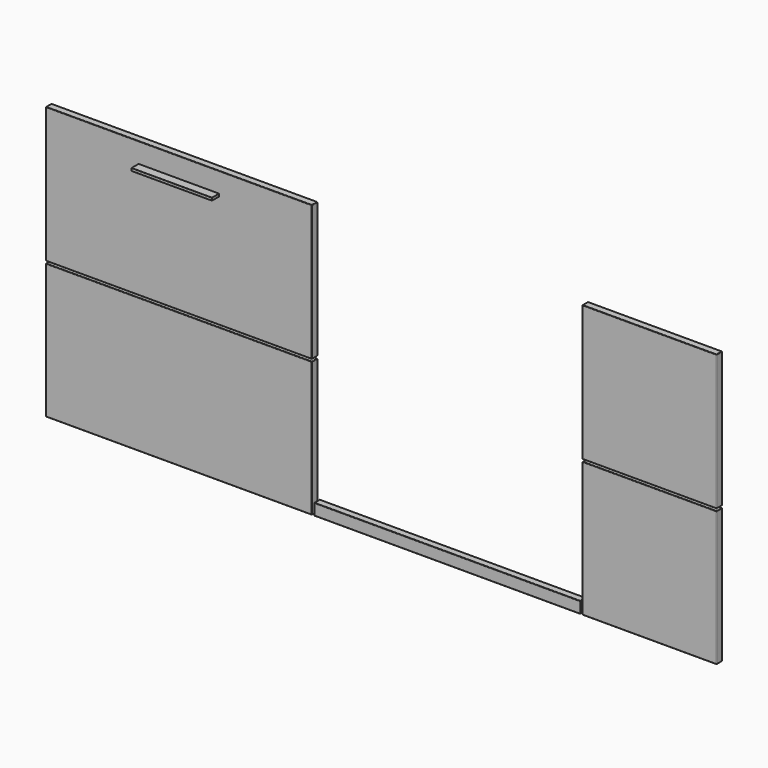
from build123d import *

# Parameters (mm, degrees)
F0_W     = 381
F0_H     = 774.7
F1_DEPTH = 19.05
F0_W_2   = 755.65
F0_H_2   = 32.6746147394
F3_W     = 228.6
F3_H     = 7.62
F4_DEPTH = 25.4
F5_R     = 0.3175
F6_W     = 2032
F6_H     = 6.35
F7_DEPTH = 25.4
F8_R     = 1.27
F8_2_R   = 1.27
F8_3_R   = 1.27


# Not quite as in the source:
# - a feature of the source that left no trace in its solid (it failed there, or was rolled back) is left out


with BuildPart() as f1:
    # F0 (on Front) → F1 (new body)
    with BuildSketch(Plane.XZ):
        with Locations((-190.5, 469.9)):
            Rectangle(F0_W, F0_H)
    extrude(amount=F1_DEPTH)


with BuildPart() as f1b:
    # F0 (on Front) → F1, piece 2 (new body)
    with BuildSketch(Plane.XZ):
        Polygon((-1904.895815666, 857.25), (-1904.9897383738, 82.4946576853), (-1149.3540530003, 82.4946576853), (-1149.3540530003, 82.55), (-1149.3540530003, 857.25), (-1527.1790530003, 857.25), align=None)
    extrude(amount=F1_DEPTH)


with BuildPart() as f1c:
    # F0 (on Front) → F1, piece 3 (new body)
    with BuildSketch(Plane.XZ):
        with Locations((-765.1790530003, 98.8873073697)):
            Rectangle(F0_W_2, F0_H_2)
    extrude(amount=F1_DEPTH)

    # F8#3
    f8_3_edges = [f1c.edges().sort_by_distance(p)[0] for p in [
        (-1143.004053, -9.525, 82.55),
        (-387.354053, -9.525, 82.55),
        (-765.179053, -19.05, 82.55),
        (-387.354053, -9.525, 115.224615),
        (-387.354053, -19.05, 98.887307),
        (-1143.004053, -9.525, 115.224615),
        (-765.179053, -19.05, 115.224615),
        (-1143.004053, -19.05, 98.887307),
    ]]
    fillet(f8_3_edges, radius=F8_3_R)


with BuildPart() as f4:
    # F3 (on face) → F4 (new body)
    with BuildSketch(Plane.XZ.offset(19.05)):
        with Locations((-1527.1250113088, 796.6017127037)):
            Rectangle(F3_W, F3_H)
    extrude(amount=F4_DEPTH)

    # F5
    f5_edges = [f4.edges().sort_by_distance(p)[0] for p in [
        (-1527.125011, -44.45, 792.791713),
        (-1412.825011, -44.45, 796.601713),
        (-1527.125011, -44.45, 800.411713),
        (-1641.425011, -44.45, 796.601713),
        (-1641.425011, -31.75, 800.411713),
        (-1641.425011, -31.75, 792.791713),
        (-1527.125011, -19.05, 800.411713),
        (-1641.425011, -19.05, 796.601713),
        (-1527.125011, -19.05, 792.791713),
        (-1412.825011, -31.75, 792.791713),
        (-1412.825011, -31.75, 800.411713),
        (-1412.825011, -19.05, 796.601713),
    ]]
    fillet(f5_edges, radius=F5_R)


with BuildPart() as f7_tool:
    # F6 (on face) → F7 (new body)
    with BuildSketch(Plane.XZ.offset(19.05)):
        with Locations((-895.2655443497, 468.8719840575)):
            Rectangle(F6_W, F6_H)
    extrude(amount=-F7_DEPTH)


with BuildPart() as f1_1:
    add(f1.part)

    # F7: cut by f7_tool
    add(f7_tool.part, mode=Mode.SUBTRACT)

    # F8
    f8_edges = [f1_1.edges().sort_by_distance(p)[0] for p in [
        (-381, -9.525, 472.046984),
        (-381, -9.525, 465.696984),
        (-381, -9.525, 82.55),
        (0, -9.525, 82.55),
        (-190.5, -19.05, 82.55),
        (-381, -19.05, 274.123492),
        (0, -9.525, 465.696984),
        (0, -19.05, 274.123492),
        (-190.5, -19.05, 465.696984),
        (-381, -19.05, 664.648492),
        (-381, -9.525, 857.25),
        (-190.5, -19.05, 472.046984),
        (0, -9.525, 472.046984),
        (-190.5, -19.05, 857.25),
        (0, -19.05, 664.648492),
        (0, -9.525, 857.25),
    ]]
    fillet(f8_edges, radius=F8_R)


with BuildPart() as f1b_1:
    add(f1b.part)

    # F7: cut by f7_tool
    add(f7_tool.part, mode=Mode.SUBTRACT)

    # F8#2
    f8_2_edges = [f1b_1.edges().sort_by_distance(p)[0] for p in [
        (-1904.942513, -9.525, 472.046984),
        (-1904.943283, -9.525, 465.696984),
        (-1904.919165, -19.05, 664.648492),
        (-1904.895816, -9.525, 857.25),
        (-1527.148283, -19.05, 472.046984),
        (-1149.354053, -9.525, 472.046984),
        (-1527.124934, -19.05, 857.25),
        (-1149.354053, -19.05, 664.648492),
        (-1149.354053, -9.525, 857.25),
        (-1904.989738, -9.525, 82.494658),
        (-1904.966511, -19.05, 274.095821),
        (-1149.354053, -9.525, 82.494658),
        (-1527.171896, -19.05, 82.494658),
        (-1527.148668, -19.05, 465.696984),
        (-1149.354053, -19.05, 274.095821),
        (-1149.354053, -9.525, 465.696984),
    ]]
    fillet(f8_2_edges, radius=F8_2_R)


solid = Compound([f1c.part, f4.part, f1_1.part, f1b_1.part])
